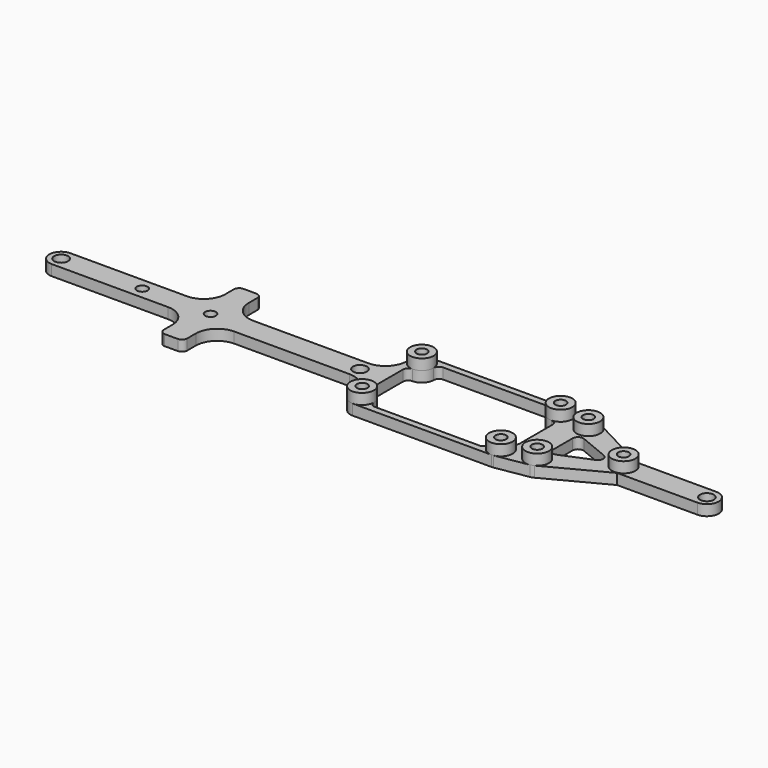
from build123d import *

# Parameters (mm, degrees)
F1_R        = 1.27
F1_R_2      = 1.651
F2_DEPTH    = 2.54
F3_R        = 2.794
F3_R_2      = 1.27
F4_DEPTH    = 2.54
F5_T1_DEPTH = 2.54
F5_T3_DEPTH = 8.8948287418
F6_R        = 5.08


# Not quite as in the source:
# - a fillet or chamfer that OpenCascade refuses, or shapes differently, is made with other operations: its cross-section is extruded or revolved along the edge and cut away or added


with BuildPart() as f2:
    # F1 (on Top) → F2 (new body)
    with BuildSketch(Plane.XY):
        with BuildLine():
            ThreePointArc((-16.51, 11.684), (-18.4856563466, 10.8656563466), (-19.304, 8.89))
            Line((-19.304, 8.89), (-19.304, 2.794))
            Line((-19.304, 2.794), (-24.13, 2.794))
            Line((-24.13, 2.794), (-56.896, 2.794))
            Line((-56.896, 2.794), (-56.896, 11.684))
            Line((-56.896, 11.684), (-62.484, 11.684))
            Line((-62.484, 11.684), (-62.484, 2.794))
            Line((-62.484, 2.794), (-95.25, 2.794))
            ThreePointArc((-95.25, 2.794), (-98.044, 0), (-95.25, -2.794))
            Line((-95.25, -2.794), (-62.484, -2.794))
            Line((-62.484, -2.794), (-62.484, -11.684))
            Line((-62.484, -11.684), (-56.896, -11.684))
            Line((-56.896, -11.684), (-56.896, -2.794))
            Line((-56.896, -2.794), (-24.13, -2.794))
            Line((-24.13, -2.794), (-19.304, -2.794))
            Line((-19.304, -2.794), (-19.304, -8.89))
            ThreePointArc((-19.304, -8.89), (-18.4856563466, -10.8656563466), (-16.51, -11.684))
            Line((-16.51, -11.684), (16.51, -11.684))
            ThreePointArc((16.51, -11.684), (16.7404506051, -11.6744799368), (16.9693307705, -11.6459846232))
            Line((16.9693307705, -11.6459846232), (24.5893307705, -10.3759846232))
            ThreePointArc((24.5893307705, -10.3759846232), (25.0216544083, -10.2679026448), (25.4312955333, -10.0924615133))
            Line((25.4312955333, -10.0924615133), (39.2983724087, -2.794))
            Line((39.2983724087, -2.794), (58.42, -2.794))
            ThreePointArc((58.42, -2.794), (61.214, 0), (58.42, 2.794))
            Line((58.42, 2.794), (39.2983724087, 2.794))
            Line((39.2983724087, 2.794), (25.4312955333, 10.0924615133))
            ThreePointArc((25.4312955333, 10.0924615133), (25.0216544083, 10.2679026448), (24.5893307705, 10.3759846232))
            Line((24.5893307705, 10.3759846232), (16.9693307705, 11.6459846232))
            ThreePointArc((16.9693307705, 11.6459846232), (16.7404506051, 11.6744799368), (16.51, 11.684))
            Line((16.51, 11.684), (-16.51, 11.684))
        make_face()
        with Locations((-16.51, -8.89)):
            Circle(F1_R, mode=Mode.SUBTRACT)
        with Locations((16.51, -8.89)):
            Circle(F1_R, mode=Mode.SUBTRACT)
        with Locations((24.13, -7.62)):
            Circle(F1_R, mode=Mode.SUBTRACT)
        with Locations((-95.25, 0)):
            Circle(F1_R_2, mode=Mode.SUBTRACT)
        with Locations((-75.946, 0)):
            Circle(F1_R, mode=Mode.SUBTRACT)
        with Locations((-59.69, 0)):
            Circle(F1_R, mode=Mode.SUBTRACT)
        with Locations((-24.13, 0)):
            Circle(F1_R_2, mode=Mode.SUBTRACT)
        with BuildLine():
            Line((-17.78, -6.4013184213), (-17.78, 6.4013184213))
            ThreePointArc((-17.78, 6.4013184213), (-14.5343436534, 6.9143436534), (-14.0213184213, 10.16))
            Line((-14.0213184213, 10.16), (14.0213184213, 10.16))
            ThreePointArc((14.0213184213, 10.16), (14.5343436534, 6.9143436534), (17.78, 6.4013184213))
            Line((17.78, 6.4013184213), (17.78, -6.4013184213))
            ThreePointArc((17.78, -6.4013184213), (14.5343436534, -6.9143436534), (14.0213184213, -10.16))
            Line((14.0213184213, -10.16), (-14.0213184213, -10.16))
            ThreePointArc((-14.0213184213, -10.16), (-14.5343436534, -6.9143436534), (-17.78, -6.4013184213))
        make_face(mode=Mode.SUBTRACT)
        Polygon((24.13, -4.826), (24.13, 4.826), (35.814, 0), align=None, mode=Mode.SUBTRACT)
        with Locations((38.608, 0)):
            Circle(F1_R, mode=Mode.SUBTRACT)
        with Locations((58.42, 0)):
            Circle(F1_R_2, mode=Mode.SUBTRACT)
        with Locations((-16.51, 8.89)):
            Circle(F1_R, mode=Mode.SUBTRACT)
        with Locations((16.51, 8.89)):
            Circle(F1_R, mode=Mode.SUBTRACT)
        with Locations((24.13, 7.62)):
            Circle(F1_R, mode=Mode.SUBTRACT)
    extrude(amount=F2_DEPTH)

    # F3 (on face) → F4 (join)
    with BuildSketch(Plane.XY.offset(2.54)):
        with Locations((-16.51, 8.89)):
            Circle(F3_R)
        with Locations((-16.51, 8.89)):
            Circle(F3_R_2, mode=Mode.SUBTRACT)
        with Locations((-16.51, -8.89)):
            Circle(F3_R)
        with Locations((-16.51, -8.89)):
            Circle(F3_R_2, mode=Mode.SUBTRACT)
        with Locations((16.51, 8.89)):
            Circle(F3_R)
        with Locations((16.51, 8.89)):
            Circle(F3_R_2, mode=Mode.SUBTRACT)
        with Locations((16.51, -8.89)):
            Circle(F3_R)
        with Locations((16.51, -8.89)):
            Circle(F3_R_2, mode=Mode.SUBTRACT)
        with Locations((24.13, 7.62)):
            Circle(F3_R)
        with Locations((24.13, 7.62)):
            Circle(F3_R_2, mode=Mode.SUBTRACT)
        with Locations((24.13, -7.62)):
            Circle(F3_R)
        with Locations((24.13, -7.62)):
            Circle(F3_R_2, mode=Mode.SUBTRACT)
        with Locations((38.608, 0)):
            Circle(F3_R)
        with Locations((38.608, 0)):
            Circle(F3_R_2, mode=Mode.SUBTRACT)
    extrude(amount=F4_DEPTH)

    # F5: fillet of radius 1.27 on 15 edges, made by hand

    # F5_s2 → F5_t1 (join)
    with BuildSketch(Plane.XY):
        with BuildLine():
            ThreePointArc((12.4455627954, 10.1604), (13.3441320819, 9.7882287264), (13.7164000162, 8.889699481))
            Line((13.7164000162, 8.889699481), (13.8434837382, 8.8897131519))
            ThreePointArc((13.8434837382, 8.8897131519), (13.9169420749, 9.5132920875), (14.1345148852, 10.1022346714))
            Line((14.1345148852, 10.1022346714), (14.0213184213, 10.2870837228))
            ThreePointArc((14.0213184213, 10.2870837228), (13.2334406084, 10.2870837228), (12.4455627954, 10.2874837228))
            Line((12.4455627954, 10.2874837228), (12.4455627954, 10.1604))
        make_face()
        with BuildLine():
            ThreePointArc((-17.7804, 4.8255627954), (-17.4082287264, 5.7241320819), (-16.509699481, 6.0964000162))
            Line((-16.509699481, 6.0964000162), (-16.5097131519, 6.2234837382))
            ThreePointArc((-16.5097131519, 6.2234837382), (-17.1332920875, 6.2969420748), (-17.7222346714, 6.5145148852))
            Line((-17.7222346714, 6.5145148852), (-17.9070837228, 6.4013184213))
            ThreePointArc((-17.9070837228, 6.4013184213), (-17.9070837228, 5.6134406084), (-17.9074837228, 4.8255627954))
            Line((-17.9074837228, 4.8255627954), (-17.7804, 4.8255627954))
        make_face()
        with BuildLine():
            ThreePointArc((-12.4455627954, 10.1604), (-13.3441320819, 9.7882287264), (-13.7164000162, 8.889699481))
            Line((-13.7164000162, 8.889699481), (-13.8434837382, 8.8897131519))
            ThreePointArc((-13.8434837382, 8.8897131519), (-13.9169420748, 9.5132920875), (-14.1345148852, 10.1022346714))
            Line((-14.1345148852, 10.1022346714), (-14.0213184213, 10.2870837228))
            ThreePointArc((-14.0213184213, 10.2870837228), (-13.2334406084, 10.2870837228), (-12.4455627954, 10.2874837228))
            Line((-12.4455627954, 10.2874837228), (-12.4455627954, 10.1604))
        make_face()
        with BuildLine():
            ThreePointArc((-12.4455627954, -10.1604), (-13.3441320819, -9.7882287264), (-13.7164000162, -8.889699481))
            Line((-13.7164000162, -8.889699481), (-13.8434837382, -8.8897131519))
            ThreePointArc((-13.8434837382, -8.8897131519), (-13.9169420748, -9.5132920875), (-14.1345148852, -10.1022346714))
            Line((-14.1345148852, -10.1022346714), (-14.0213184213, -10.2870837228))
            ThreePointArc((-14.0213184213, -10.2870837228), (-13.2334406084, -10.2870837228), (-12.4455627954, -10.2874837228))
            Line((-12.4455627954, -10.2874837228), (-12.4455627954, -10.1604))
        make_face()
        with BuildLine():
            ThreePointArc((-17.7804, -4.8255627954), (-17.4082287264, -5.7241320819), (-16.509699481, -6.0964000162))
            Line((-16.509699481, -6.0964000162), (-16.5097131519, -6.2234837382))
            ThreePointArc((-16.5097131519, -6.2234837382), (-17.1332920875, -6.2969420748), (-17.7222346714, -6.5145148852))
            Line((-17.7222346714, -6.5145148852), (-17.9070837228, -6.4013184213))
            ThreePointArc((-17.9070837228, -6.4013184213), (-17.9070837228, -5.6134406084), (-17.9074837228, -4.8255627954))
            Line((-17.9074837228, -4.8255627954), (-17.7804, -4.8255627954))
        make_face()
        with BuildLine():
            ThreePointArc((13.7164000162, -8.889699481), (13.3441320819, -9.7882287264), (12.4455627954, -10.1604))
            Line((12.4455627954, -10.1604), (12.4455627954, -10.2874837228))
            ThreePointArc((12.4455627954, -10.2874837228), (13.2334406084, -10.2870837228), (14.0213184213, -10.2870837228))
            Line((14.0213184213, -10.2870837228), (14.1345148852, -10.1022346714))
            ThreePointArc((14.1345148852, -10.1022346714), (13.9169420748, -9.5132920875), (13.8434837382, -8.8897131519))
            Line((13.8434837382, -8.8897131519), (13.7164000162, -8.889699481))
        make_face()
        with BuildLine():
            ThreePointArc((16.509699481, -6.0964000162), (17.4082287264, -5.7241320819), (17.7804, -4.8255627954))
            Line((17.7804, -4.8255627954), (17.9074837228, -4.8255627954))
            ThreePointArc((17.9074837228, -4.8255627954), (17.9070837228, -5.6134406084), (17.9070837228, -6.4013184213))
            Line((17.9070837228, -6.4013184213), (17.7222346714, -6.5145148852))
            ThreePointArc((17.7222346714, -6.5145148852), (17.1332920875, -6.2969420748), (16.5097131519, -6.2234837382))
            Line((16.5097131519, -6.2234837382), (16.509699481, -6.0964000162))
        make_face()
        with BuildLine():
            ThreePointArc((17.7804, 4.8255627954), (17.4082287264, 5.7241320819), (16.509699481, 6.0964000162))
            Line((16.509699481, 6.0964000162), (16.5097131519, 6.2234837382))
            ThreePointArc((16.5097131519, 6.2234837382), (17.1332920875, 6.2969420749), (17.7222346714, 6.5145148852))
            Line((17.7222346714, 6.5145148852), (17.9070837228, 6.4013184213))
            ThreePointArc((17.9070837228, 6.4013184213), (17.9070837228, 5.6134406084), (17.9074837228, 4.8255627954))
            Line((17.9074837228, 4.8255627954), (17.7804, 4.8255627954))
        make_face()
        with BuildLine():
            ThreePointArc((25.8856801845, 4.1012605278), (24.6938983618, 3.9829784639), (24.1296, 2.9266158754))
            Line((24.1296, 2.9266158754), (24.0025099128, 2.9266158754))
            ThreePointArc((24.0025099128, 2.9266158754), (24.0029099128, 3.8763079377), (24.0029099128, 4.826))
            Line((24.0029099128, 4.826), (24.1785179313, 4.9434644652))
            ThreePointArc((24.1785179313, 4.9434644652), (25.0562816715, 4.5809098769), (25.9341981158, 4.2187249931))
            Line((25.9341981158, 4.2187249931), (25.8856801845, 4.1012605278))
        make_face()
        with BuildLine():
            ThreePointArc((25.8856801845, -4.1012605278), (24.6938983618, -3.9829784639), (24.1296, -2.9266158754))
            Line((24.1296, -2.9266158754), (24.0025099128, -2.9266158754))
            ThreePointArc((24.0025099128, -2.9266158754), (24.0029099128, -3.8763079377), (24.0029099128, -4.826))
            Line((24.0029099128, -4.826), (24.1785179313, -4.9434644652))
            ThreePointArc((24.1785179313, -4.9434644652), (25.0562816715, -4.5809098769), (25.9341981158, -4.2187249931))
            Line((25.9341981158, -4.2187249931), (25.8856801845, -4.1012605278))
        make_face()
        with BuildLine():
            ThreePointArc((32.9717393402, -1.174410007), (33.7573039441, 0), (32.9717393402, 1.174410007))
            Line((32.9717393402, 1.174410007), (33.0202475797, 1.2918510077))
            ThreePointArc((33.0202475797, 1.2918510077), (34.4413015575, 0.7044611519), (35.8625082394, 0.1174410007))
            Line((35.8625082394, 0.1174410007), (35.8625082394, -0.1174410007))
            ThreePointArc((35.8625082394, -0.1174410007), (34.4413015575, -0.7044611519), (33.0202475797, -1.2918510077))
            Line((33.0202475797, -1.2918510077), (32.9717393402, -1.174410007))
        make_face()
    extrude(amount=F5_T1_DEPTH)

    # F5_s4 → F5_t3 (cut)
    with BuildSketch(Plane.XY.offset(-3.1774143709)):
        with BuildLine():
            ThreePointArc((-61.2130343146, 11.6844), (-62.1120256121, 11.3120256121), (-62.4844, 10.4130343146))
            Line((-62.4844, 10.4130343146), (-62.6115365685, 10.4130343146))
            ThreePointArc((-62.6115365685, 10.4130343146), (-62.6111365685, 11.0485171573), (-62.6111365685, 11.684))
            Line((-62.6111365685, 11.684), (-62.484, 11.8111365685))
            ThreePointArc((-62.484, 11.8111365685), (-61.8485171573, 11.8111365685), (-61.2130343146, 11.8115365685))
            Line((-61.2130343146, 11.8115365685), (-61.2130343146, 11.6844))
        make_face()
        with BuildLine():
            ThreePointArc((-58.1669656854, -11.6844), (-57.2679743879, -11.3120256121), (-56.8956, -10.4130343146))
            Line((-56.8956, -10.4130343146), (-56.7684634315, -10.4130343146))
            ThreePointArc((-56.7684634315, -10.4130343146), (-56.7688634315, -11.0485171573), (-56.7688634315, -11.684))
            Line((-56.7688634315, -11.684), (-56.896, -11.8111365685))
            ThreePointArc((-56.896, -11.8111365685), (-57.5314828427, -11.8111365685), (-58.1669656854, -11.8115365685))
            Line((-58.1669656854, -11.8115365685), (-58.1669656854, -11.6844))
        make_face()
        with BuildLine():
            ThreePointArc((-62.4844, -10.4130343146), (-62.1120256121, -11.3120256121), (-61.2130343146, -11.6844))
            Line((-61.2130343146, -11.6844), (-61.2130343146, -11.8115365685))
            ThreePointArc((-61.2130343146, -11.8115365685), (-61.8485171573, -11.8111365685), (-62.484, -11.8111365685))
            Line((-62.484, -11.8111365685), (-62.6111365685, -11.684))
            ThreePointArc((-62.6111365685, -11.684), (-62.6111365685, -11.0485171573), (-62.6115365685, -10.4130343146))
            Line((-62.6115365685, -10.4130343146), (-62.4844, -10.4130343146))
        make_face()
        with BuildLine():
            ThreePointArc((-56.8956, 10.4130343146), (-57.2679743879, 11.3120256121), (-58.1669656854, 11.6844))
            Line((-58.1669656854, 11.6844), (-58.1669656854, 11.8115365685))
            ThreePointArc((-58.1669656854, 11.8115365685), (-57.5314828427, 11.8111365685), (-56.896, 11.8111365685))
            Line((-56.896, 11.8111365685), (-56.7688634315, 11.684))
            ThreePointArc((-56.7688634315, 11.684), (-56.7688634315, 11.0485171573), (-56.7684634315, 10.4130343146))
            Line((-56.7684634315, 10.4130343146), (-56.8956, 10.4130343146))
        make_face()
    extrude(amount=F5_T3_DEPTH, mode=Mode.SUBTRACT)

    # F6
    f6_edges = [f2.edges().sort_by_distance(p)[0] for p in [
        (-62.484, 2.794, 1.27),
        (-19.304, 2.794, 1.27),
        (-62.484, -2.794, 1.27),
        (-56.896, -2.794, 1.27),
        (-56.896, 2.794, 1.27),
        (-19.304, -2.794, 1.27),
    ]]
    fillet(f6_edges, radius=F6_R)


solid = f2.part
